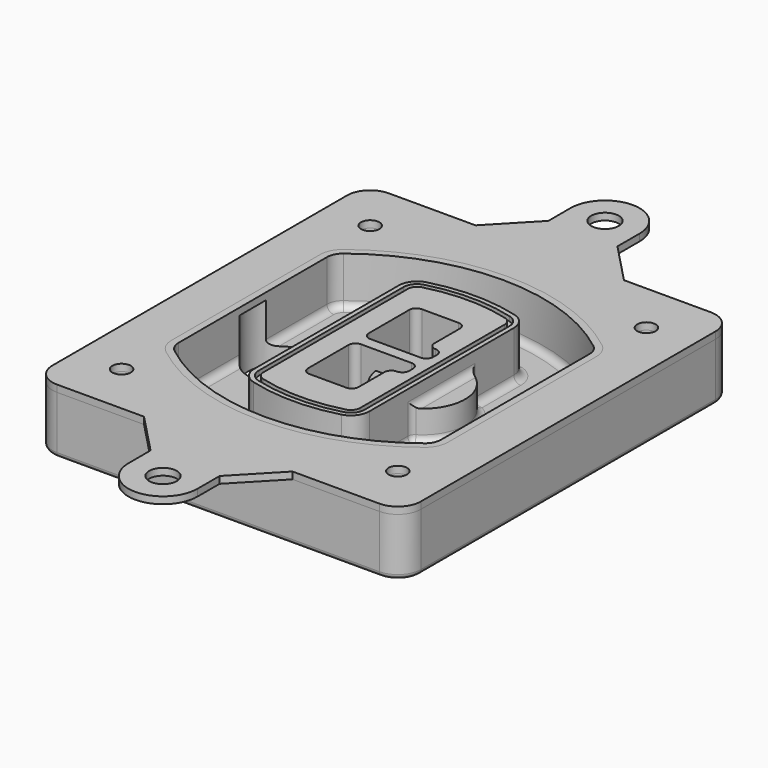
from build123d import *

# Parameters (mm, degrees)
F0_R      = 4
F1_DEPTH  = 25
F2_DEPTH  = 3
F3_DEPTH  = 18
F5_DEPTH  = 21
F6_DEPTH  = 2
F8_DEPTH  = 20
F9_DEPTH  = 16
F10_DEPTH = 25
F7_R      = 6
F7_R_2    = 4
F11_DEPTH = 6
F13_DEPTH = 9
F14_R     = 3
F15_R     = 2
F16_R     = 6
F16_R_2   = 4
F17_DEPTH = 3


with BuildPart() as f1:
    # F0 (on Top) → F1 (new body)
    with BuildSketch(Plane.XY):
        with BuildLine():
            ThreePointArc((-80, -80), (-77.0710678119, -87.0710678119), (-70, -90))
            Line((-70, -90), (70, -90))
            ThreePointArc((70, -90), (77.0710678119, -87.0710678119), (80, -80))
            Line((80, -80), (80, 80))
            ThreePointArc((80, 80), (77.0710678119, 87.0710678119), (70, 90))
            Line((70, 90), (-70, 90))
            ThreePointArc((-70, 90), (-77.0710678119, 87.0710678119), (-80, 80))
            Line((-80, 80), (-80, -80))
        make_face()
        with Locations((-60, -67.5)):
            Circle(F0_R, mode=Mode.SUBTRACT)
        with Locations((60, -67.5)):
            Circle(F0_R, mode=Mode.SUBTRACT)
        with Locations((-60, 67.5)):
            Circle(F0_R, mode=Mode.SUBTRACT)
        with BuildLine():
            ThreePointArc((-64, 40.2934422872), (-62.5820384798, 46.4328484224), (-58.6153846154, 51.3286200352))
            ThreePointArc((-58.6153846154, 51.3286200352), (0, 71.5), (58.6153846154, 51.3286200352))
            ThreePointArc((58.6153846154, 51.3286200352), (62.5820384798, 46.4328484224), (64, 40.2934422872))
            Line((64, 40.2934422872), (64, -40.2934422872))
            ThreePointArc((64, -40.2934422872), (62.5820384798, -46.4328484224), (58.6153846154, -51.3286200352))
            ThreePointArc((58.6153846154, -51.3286200352), (0, -71.5), (-58.6153846154, -51.3286200352))
            ThreePointArc((-58.6153846154, -51.3286200352), (-62.5820384798, -46.4328484224), (-64, -40.2934422872))
            Line((-64, -40.2934422872), (-64, 40.2934422872))
        make_face(mode=Mode.SUBTRACT)
        with Locations((60, 67.5)):
            Circle(F0_R, mode=Mode.SUBTRACT)
        with BuildLine():
            ThreePointArc((58.6153846154, 51.3286200352), (0, 71.5), (-58.6153846154, 51.3286200352))
            ThreePointArc((-58.6153846154, 51.3286200352), (-62.5820384798, 46.4328484224), (-64, 40.2934422872))
            Line((-64, 40.2934422872), (-64, -40.2934422872))
            ThreePointArc((-64, -40.2934422872), (-62.5820384798, -46.4328484224), (-58.6153846154, -51.3286200352))
            ThreePointArc((-58.6153846154, -51.3286200352), (0, -71.5), (58.6153846154, -51.3286200352))
            ThreePointArc((58.6153846154, -51.3286200352), (62.5820384798, -46.4328484224), (64, -40.2934422872))
            Line((64, -40.2934422872), (64, 40.2934422872))
            ThreePointArc((64, 40.2934422872), (62.5820384798, 46.4328484224), (58.6153846154, 51.3286200352))
        make_face()
        with BuildLine():
            Line((-60, -40.2934422872), (-60, 40.2934422872))
            ThreePointArc((-60, 40.2934422872), (-58.9871703427, 44.6787323838), (-56.1538461538, 48.1757121072))
            ThreePointArc((-56.1538461538, 48.1757121072), (0, 67.5), (56.1538461538, 48.1757121072))
            ThreePointArc((56.1538461538, 48.1757121072), (58.9871703427, 44.6787323838), (60, 40.2934422872))
            Line((60, 40.2934422872), (60, -40.2934422872))
            ThreePointArc((60, -40.2934422872), (58.9871703427, -44.6787323838), (56.1538461538, -48.1757121072))
            ThreePointArc((56.1538461538, -48.1757121072), (0, -67.5), (-56.1538461538, -48.1757121072))
            ThreePointArc((-56.1538461538, -48.1757121072), (-58.9871703427, -44.6787323838), (-60, -40.2934422872))
        make_face(mode=Mode.SUBTRACT)
        with BuildLine():
            ThreePointArc((-56.1538461538, 48.1757121072), (-58.9871703427, 44.6787323838), (-60, 40.2934422872))
            Line((-60, 40.2934422872), (-60, -40.2934422872))
            ThreePointArc((-60, -40.2934422872), (-58.9871703427, -44.6787323838), (-56.1538461538, -48.1757121072))
            ThreePointArc((-56.1538461538, -48.1757121072), (0, -67.5), (56.1538461538, -48.1757121072))
            ThreePointArc((56.1538461538, -48.1757121072), (58.9871703427, -44.6787323838), (60, -40.2934422872))
            Line((60, -40.2934422872), (60, 40.2934422872))
            ThreePointArc((60, 40.2934422872), (58.9871703427, 44.6787323838), (56.1538461538, 48.1757121072))
            ThreePointArc((56.1538461538, 48.1757121072), (0, 67.5), (-56.1538461538, 48.1757121072))
        make_face()
        with BuildLine():
            ThreePointArc((54.3076923077, 45.8110311612), (56.2910192399, 43.3631453548), (57, 40.2934422872))
            Line((57, 40.2934422872), (57, -40.2934422872))
            ThreePointArc((57, -40.2934422872), (56.2910192399, -43.3631453548), (54.3076923077, -45.8110311612))
            ThreePointArc((54.3076923077, -45.8110311612), (0, -64.5), (-54.3076923077, -45.8110311612))
            ThreePointArc((-54.3076923077, -45.8110311612), (-56.2910192399, -43.3631453548), (-57, -40.2934422872))
            Line((-57, -40.2934422872), (-57, 40.2934422872))
            ThreePointArc((-57, 40.2934422872), (-56.2910192399, 43.3631453548), (-54.3076923077, 45.8110311612))
            ThreePointArc((-54.3076923077, 45.8110311612), (0, 64.5), (54.3076923077, 45.8110311612))
        make_face(mode=Mode.SUBTRACT)
        with BuildLine():
            Line((57, -40.2934422872), (57, 40.2934422872))
            ThreePointArc((57, 40.2934422872), (56.2910192399, 43.3631453548), (54.3076923077, 45.8110311612))
            ThreePointArc((54.3076923077, 45.8110311612), (0, 64.5), (-54.3076923077, 45.8110311612))
            ThreePointArc((-54.3076923077, 45.8110311612), (-56.2910192399, 43.3631453548), (-57, 40.2934422872))
            Line((-57, 40.2934422872), (-57, -40.2934422872))
            ThreePointArc((-57, -40.2934422872), (-56.2910192399, -43.3631453548), (-54.3076923077, -45.8110311612))
            ThreePointArc((-54.3076923077, -45.8110311612), (0, -64.5), (54.3076923077, -45.8110311612))
            ThreePointArc((54.3076923077, -45.8110311612), (56.2910192399, -43.3631453548), (57, -40.2934422872))
        make_face()
    extrude(amount=-F1_DEPTH)

    # F0 (on Top) → F2 (join)
    with BuildSketch(Plane.XY):
        with BuildLine():
            ThreePointArc((-56.1538461538, 48.1757121072), (-58.9871703427, 44.6787323838), (-60, 40.2934422872))
            Line((-60, 40.2934422872), (-60, -40.2934422872))
            ThreePointArc((-60, -40.2934422872), (-58.9871703427, -44.6787323838), (-56.1538461538, -48.1757121072))
            ThreePointArc((-56.1538461538, -48.1757121072), (0, -67.5), (56.1538461538, -48.1757121072))
            ThreePointArc((56.1538461538, -48.1757121072), (58.9871703427, -44.6787323838), (60, -40.2934422872))
            Line((60, -40.2934422872), (60, 40.2934422872))
            ThreePointArc((60, 40.2934422872), (58.9871703427, 44.6787323838), (56.1538461538, 48.1757121072))
            ThreePointArc((56.1538461538, 48.1757121072), (0, 67.5), (-56.1538461538, 48.1757121072))
        make_face()
        with BuildLine():
            ThreePointArc((54.3076923077, 45.8110311612), (56.2910192399, 43.3631453548), (57, 40.2934422872))
            Line((57, 40.2934422872), (57, -40.2934422872))
            ThreePointArc((57, -40.2934422872), (56.2910192399, -43.3631453548), (54.3076923077, -45.8110311612))
            ThreePointArc((54.3076923077, -45.8110311612), (0, -64.5), (-54.3076923077, -45.8110311612))
            ThreePointArc((-54.3076923077, -45.8110311612), (-56.2910192399, -43.3631453548), (-57, -40.2934422872))
            Line((-57, -40.2934422872), (-57, 40.2934422872))
            ThreePointArc((-57, 40.2934422872), (-56.2910192399, 43.3631453548), (-54.3076923077, 45.8110311612))
            ThreePointArc((-54.3076923077, 45.8110311612), (0, 64.5), (54.3076923077, 45.8110311612))
        make_face(mode=Mode.SUBTRACT)
    extrude(amount=F2_DEPTH)

    # F0 (on Top) → F3 (cut)
    with BuildSketch(Plane.XY):
        with BuildLine():
            Line((57, -40.2934422872), (57, 40.2934422872))
            ThreePointArc((57, 40.2934422872), (56.2910192399, 43.3631453548), (54.3076923077, 45.8110311612))
            ThreePointArc((54.3076923077, 45.8110311612), (0, 64.5), (-54.3076923077, 45.8110311612))
            ThreePointArc((-54.3076923077, 45.8110311612), (-56.2910192399, 43.3631453548), (-57, 40.2934422872))
            Line((-57, 40.2934422872), (-57, -40.2934422872))
            ThreePointArc((-57, -40.2934422872), (-56.2910192399, -43.3631453548), (-54.3076923077, -45.8110311612))
            ThreePointArc((-54.3076923077, -45.8110311612), (0, -64.5), (54.3076923077, -45.8110311612))
            ThreePointArc((54.3076923077, -45.8110311612), (56.2910192399, -43.3631453548), (57, -40.2934422872))
        make_face()
    extrude(amount=-F3_DEPTH, mode=Mode.SUBTRACT)

    # F4 (on face) → F5 (join, through all)
    with BuildSketch(Plane.XY.offset(3)):
        with BuildLine():
            ThreePointArc((-25, -39.2465276821), (-23.3511545998, -44.1109737193), (-19.0842911877, -46.9702398883))
            ThreePointArc((-19.0842911877, -46.9702398883), (0, -49.5), (19.0842911877, -46.9702398883))
            ThreePointArc((19.0842911877, -46.9702398883), (23.3511545998, -44.1109737193), (25, -39.2465276821))
            Line((25, -39.2465276821), (25, 39.2465276821))
            ThreePointArc((25, 39.2465276821), (23.3511545998, 44.1109737193), (19.0842911877, 46.9702398883))
            ThreePointArc((19.0842911877, 46.9702398883), (0, 49.5), (-19.0842911877, 46.9702398883))
            ThreePointArc((-19.0842911877, 46.9702398883), (-23.3511545998, 44.1109737193), (-25, 39.2465276821))
            Line((-25, 39.2465276821), (-25, -39.2465276821))
        make_face()
        with BuildLine():
            ThreePointArc((18.5632183908, 45.0393118368), (21.7633659499, 42.89486221), (23, 39.2465276821))
            Line((23, 39.2465276821), (23, -39.2465276821))
            ThreePointArc((23, -39.2465276821), (21.7633659499, -42.89486221), (18.5632183908, -45.0393118368))
            ThreePointArc((18.5632183908, -45.0393118368), (0, -47.5), (-18.5632183908, -45.0393118368))
            ThreePointArc((-18.5632183908, -45.0393118368), (-21.7633659499, -42.89486221), (-23, -39.2465276821))
            Line((-23, -39.2465276821), (-23, 39.2465276821))
            ThreePointArc((-23, 39.2465276821), (-21.7633659499, 42.89486221), (-18.5632183908, 45.0393118368))
            ThreePointArc((-18.5632183908, 45.0393118368), (0, 47.5), (18.5632183908, 45.0393118368))
        make_face(mode=Mode.SUBTRACT)
        with BuildLine():
            Line((23, -39.2465276821), (23, 39.2465276821))
            ThreePointArc((23, 39.2465276821), (21.7633659499, 42.89486221), (18.5632183908, 45.0393118368))
            ThreePointArc((18.5632183908, 45.0393118368), (0, 47.5), (-18.5632183908, 45.0393118368))
            ThreePointArc((-18.5632183908, 45.0393118368), (-21.7633659499, 42.89486221), (-23, 39.2465276821))
            Line((-23, 39.2465276821), (-23, -39.2465276821))
            ThreePointArc((-23, -39.2465276821), (-21.7633659499, -42.89486221), (-18.5632183908, -45.0393118368))
            ThreePointArc((-18.5632183908, -45.0393118368), (0, -47.5), (18.5632183908, -45.0393118368))
            ThreePointArc((18.5632183908, -45.0393118368), (21.7633659499, -42.89486221), (23, -39.2465276821))
        make_face()
        with BuildLine():
            ThreePointArc((18.0421455939, 43.1083837852), (20.1755772999, 41.6787507007), (21, 39.2465276821))
            Line((21, 39.2465276821), (21, -39.2465276821))
            ThreePointArc((21, -39.2465276821), (20.1755772999, -41.6787507007), (18.0421455939, -43.1083837852))
            ThreePointArc((18.0421455939, -43.1083837852), (0, -45.5), (-18.0421455939, -43.1083837852))
            ThreePointArc((-18.0421455939, -43.1083837852), (-20.1755772999, -41.6787507007), (-21, -39.2465276821))
            Line((-21, -39.2465276821), (-21, 39.2465276821))
            ThreePointArc((-21, 39.2465276821), (-20.1755772999, 41.6787507007), (-18.0421455939, 43.1083837852))
            ThreePointArc((-18.0421455939, 43.1083837852), (0, 45.5), (18.0421455939, 43.1083837852))
        make_face(mode=Mode.SUBTRACT)
        with BuildLine():
            Line((21, -39.2465276821), (21, 39.2465276821))
            ThreePointArc((21, 39.2465276821), (20.1755772999, 41.6787507007), (18.0421455939, 43.1083837852))
            ThreePointArc((18.0421455939, 43.1083837852), (0, 45.5), (-18.0421455939, 43.1083837852))
            ThreePointArc((-18.0421455939, 43.1083837852), (-20.1755772999, 41.6787507007), (-21, 39.2465276821))
            Line((-21, 39.2465276821), (-21, -39.2465276821))
            ThreePointArc((-21, -39.2465276821), (-20.1755772999, -41.6787507007), (-18.0421455939, -43.1083837852))
            ThreePointArc((-18.0421455939, -43.1083837852), (0, -45.5), (18.0421455939, -43.1083837852))
            ThreePointArc((18.0421455939, -43.1083837852), (20.1755772999, -41.6787507007), (21, -39.2465276821))
        make_face()
        with BuildLine():
            Line((-8, -2.5), (14, -2.5))
            ThreePointArc((14, -2.5), (16.1213203436, -3.3786796564), (17, -5.5))
            Line((17, -5.5), (17, -7.5))
            ThreePointArc((17, -7.5), (16.1213203436, -9.6213203436), (14, -10.5))
            ThreePointArc((14, -10.5), (11.8786796564, -11.3786796564), (11, -13.5))
            Line((11, -13.5), (11, -27.5))
            ThreePointArc((11, -27.5), (10.1213203436, -29.6213203436), (8, -30.5))
            Line((8, -30.5), (-8, -30.5))
            ThreePointArc((-8, -30.5), (-10.1213203436, -29.6213203436), (-11, -27.5))
            Line((-11, -27.5), (-11, -5.5))
            ThreePointArc((-11, -5.5), (-10.1213203436, -3.3786796564), (-8, -2.5))
        make_face(mode=Mode.SUBTRACT)
        with BuildLine():
            ThreePointArc((-8, 2.5), (-10.1213203436, 3.3786796564), (-11, 5.5))
            Line((-11, 5.5), (-11, 27.5))
            ThreePointArc((-11, 27.5), (-10.1213203436, 29.6213203436), (-8, 30.5))
            Line((-8, 30.5), (8, 30.5))
            ThreePointArc((8, 30.5), (10.1213203436, 29.6213203436), (11, 27.5))
            Line((11, 27.5), (11, 13.5))
            ThreePointArc((11, 13.5), (11.8786796564, 11.3786796564), (14, 10.5))
            ThreePointArc((14, 10.5), (16.1213203436, 9.6213203436), (17, 7.5))
            Line((17, 7.5), (17, 5.5))
            ThreePointArc((17, 5.5), (16.1213203436, 3.3786796564), (14, 2.5))
            Line((14, 2.5), (-8, 2.5))
        make_face(mode=Mode.SUBTRACT)
    extrude(amount=-F5_DEPTH)

    # F4 (on face) → F6 (cut)
    with BuildSketch(Plane.XY.offset(3)):
        with BuildLine():
            Line((23, -39.2465276821), (23, 39.2465276821))
            ThreePointArc((23, 39.2465276821), (21.7633659499, 42.89486221), (18.5632183908, 45.0393118368))
            ThreePointArc((18.5632183908, 45.0393118368), (0, 47.5), (-18.5632183908, 45.0393118368))
            ThreePointArc((-18.5632183908, 45.0393118368), (-21.7633659499, 42.89486221), (-23, 39.2465276821))
            Line((-23, 39.2465276821), (-23, -39.2465276821))
            ThreePointArc((-23, -39.2465276821), (-21.7633659499, -42.89486221), (-18.5632183908, -45.0393118368))
            ThreePointArc((-18.5632183908, -45.0393118368), (0, -47.5), (18.5632183908, -45.0393118368))
            ThreePointArc((18.5632183908, -45.0393118368), (21.7633659499, -42.89486221), (23, -39.2465276821))
        make_face()
        with BuildLine():
            ThreePointArc((18.0421455939, 43.1083837852), (20.1755772999, 41.6787507007), (21, 39.2465276821))
            Line((21, 39.2465276821), (21, -39.2465276821))
            ThreePointArc((21, -39.2465276821), (20.1755772999, -41.6787507007), (18.0421455939, -43.1083837852))
            ThreePointArc((18.0421455939, -43.1083837852), (0, -45.5), (-18.0421455939, -43.1083837852))
            ThreePointArc((-18.0421455939, -43.1083837852), (-20.1755772999, -41.6787507007), (-21, -39.2465276821))
            Line((-21, -39.2465276821), (-21, 39.2465276821))
            ThreePointArc((-21, 39.2465276821), (-20.1755772999, 41.6787507007), (-18.0421455939, 43.1083837852))
            ThreePointArc((-18.0421455939, 43.1083837852), (0, 45.5), (18.0421455939, 43.1083837852))
        make_face(mode=Mode.SUBTRACT)
    extrude(amount=-F6_DEPTH, mode=Mode.SUBTRACT)

    # F7 (on face) → F8 (join)
    with BuildSketch(Plane(origin=(0, 0, -25), x_dir=(1, 0, 0), z_dir=(0, 0, -1))):
        with BuildLine():
            ThreePointArc((3.28842436, 0), (16.7567035675, 13.4682792075), (30.224982775, 0))
            Line((30.224982775, 0), (35.224982775, 0))
            ThreePointArc((35.224982775, 0), (16.7567035675, 18.4682792075), (-1.71157564, 0))
            Line((-1.71157564, 0), (3.28842436, 0))
        make_face()
        with BuildLine():
            Line((3.28842436, 0), (30.224982775, 0))
            ThreePointArc((30.224982775, 0), (16.7567035675, 13.4682792075), (3.28842436, 0))
        make_face()
        with BuildLine():
            ThreePointArc((3.28842436, 0), (16.7567035675, -13.4682792075), (30.224982775, 0))
            Line((30.224982775, 0), (3.28842436, 0))
        make_face()
        with BuildLine():
            Line((35.224982775, 0), (30.224982775, 0))
            ThreePointArc((30.224982775, 0), (16.7567035675, -13.4682792075), (3.28842436, 0))
            Line((3.28842436, 0), (-1.71157564, 0))
            ThreePointArc((-1.71157564, 0), (16.7567035675, -18.4682792075), (35.224982775, 0))
        make_face()
    extrude(amount=-F8_DEPTH)

    # F7 (on face) → F9 (cut)
    with BuildSketch(Plane(origin=(0, 0, -25), x_dir=(1, 0, 0), z_dir=(0, 0, -1))):
        with BuildLine():
            Line((3.28842436, 0), (30.224982775, 0))
            ThreePointArc((30.224982775, 0), (16.7567035675, 13.4682792075), (3.28842436, 0))
        make_face()
        with BuildLine():
            ThreePointArc((3.28842436, 0), (16.7567035675, -13.4682792075), (30.224982775, 0))
            Line((30.224982775, 0), (3.28842436, 0))
        make_face()
    extrude(amount=-F9_DEPTH, mode=Mode.SUBTRACT)

    # F7 (on face) → F10 (cut)
    with BuildSketch(Plane(origin=(0, 0, -25), x_dir=(1, 0, 0), z_dir=(0, 0, -1))):
        with BuildLine():
            Line((-59.0318229325, 0), (-32.0952645175, 0))
            ThreePointArc((-32.0952645175, 0), (-45.563543725, 13.4682792075), (-59.0318229325, 0))
        make_face()
        with BuildLine():
            ThreePointArc((-59.0318229325, 0), (-45.563543725, -13.4682792075), (-32.0952645175, 0))
            Line((-32.0952645175, 0), (-59.0318229325, 0))
        make_face()
    extrude(amount=-F10_DEPTH, mode=Mode.SUBTRACT)

    # F7 (on face) → F11 (cut)
    with BuildSketch(Plane(origin=(0, 0, -25), x_dir=(1, 0, 0), z_dir=(0, 0, -1))):
        with Locations((60, -67.5)):
            Circle(F7_R)
        with Locations((60, -67.5)):
            Circle(F7_R_2, mode=Mode.SUBTRACT)
        with Locations((-60, -67.5)):
            Circle(F7_R)
        with Locations((-60, -67.5)):
            Circle(F7_R_2, mode=Mode.SUBTRACT)
        with Locations((-60, 67.5)):
            Circle(F7_R)
        with Locations((-60, 67.5)):
            Circle(F7_R_2, mode=Mode.SUBTRACT)
        with Locations((60, 67.5)):
            Circle(F7_R)
        with Locations((60, 67.5)):
            Circle(F7_R_2, mode=Mode.SUBTRACT)
    extrude(amount=-F11_DEPTH, mode=Mode.SUBTRACT)

    # F12 (on face) → F13 (cut, through all)
    with BuildSketch(Plane(origin=(0, 0, -9), x_dir=(1, 0, 0), z_dir=(0, 0, -1))):
        with BuildLine():
            Line((11, 13.5), (11, 17.5481537753))
            ThreePointArc((11, 17.5481537753), (2.5696536419, 11.8239143813), (-1.5415842455, 2.5))
            Line((-1.5415842455, 2.5), (3.5224848595, 2.5))
            ThreePointArc((3.5224848595, 2.5), (6.1857188154, 8.3455872281), (11.2536447004, 12.2927168648))
            ThreePointArc((11.2536447004, 12.2927168648), (11.0640958889, 12.8831798879), (11, 13.5))
        make_face()
        with BuildLine():
            ThreePointArc((11.2536447004, -12.2927168648), (6.1857188154, -8.3455872281), (3.5224848595, -2.5))
            Line((3.5224848595, -2.5), (-1.5415842455, -2.5))
            ThreePointArc((-1.5415842455, -2.5), (2.5696536419, -11.8239143813), (11, -17.5481537753))
            Line((11, -17.5481537753), (11, -13.5))
            ThreePointArc((11, -13.5), (11.0640958889, -12.8831798879), (11.2536447004, -12.2927168648))
        make_face()
        with BuildLine():
            ThreePointArc((11.2536447004, 12.2927168648), (6.1857188154, 8.3455872281), (3.5224848595, 2.5))
            Line((3.5224848595, 2.5), (14, 2.5))
            ThreePointArc((14, 2.5), (16.1213203436, 3.3786796564), (17, 5.5))
            Line((17, 5.5), (17, 7.5))
            ThreePointArc((17, 7.5), (16.1213203436, 9.6213203436), (14, 10.5))
            ThreePointArc((14, 10.5), (12.3601599782, 10.9878446101), (11.2536447004, 12.2927168648))
        make_face()
        with BuildLine():
            Line((14, -2.5), (3.5224848595, -2.5))
            ThreePointArc((3.5224848595, -2.5), (6.1857188154, -8.3455872281), (11.2536447004, -12.2927168648))
            ThreePointArc((11.2536447004, -12.2927168648), (12.3601599782, -10.9878446101), (14, -10.5))
            ThreePointArc((14, -10.5), (16.1213203436, -9.6213203436), (17, -7.5))
            Line((17, -7.5), (17, -5.5))
            ThreePointArc((17, -5.5), (16.1213203436, -3.3786796564), (14, -2.5))
        make_face()
    extrude(amount=F13_DEPTH, mode=Mode.SUBTRACT)

    # F14
    f14_edges = [f1.edges().sort_by_distance(p)[0] for p in [
        (-57, -23.703476, -18),
        (-57, 23.703476, -18),
        (25, 0, -5),
        (25, 16.526506, -11.5),
        (25, -16.526506, -11.5),
        (25, -27.886517, -18),
        (35.224983, 0, -18),
    ]]
    fillet(f14_edges, radius=F14_R)

    # F15
    f15_edges = [f1.edges().sort_by_distance(p)[0] for p in [
        (0, -90, -25),
    ]]
    fillet(f15_edges, radius=F15_R)


with BuildPart() as f17:
    # F16 (on face) → F17 (new body, through all)
    with BuildSketch(Plane.XY):
        with BuildLine():
            Line((-32.2395451367, -90), (-15, -108))
            Line((-15, -108), (-15, -120))
            ThreePointArc((-15, -120), (0, -135), (15, -120))
            Line((15, -120), (15, -108))
            Line((15, -108), (32.2395451367, -90))
            Line((32.2395451367, -90), (-32.2395451367, -90))
        make_face()
        with Locations((0, -120)):
            Circle(F16_R, mode=Mode.SUBTRACT)
        with BuildLine():
            Line((32.2395451367, 90), (-32.2395451367, 90))
            Line((-32.2395451367, 90), (-33, 90))
            Line((-33, 90), (-70, 90))
            ThreePointArc((-70, 90), (-77.0710678119, 87.0710678119), (-80, 80))
            Line((-80, 80), (-80, -80))
            ThreePointArc((-80, -80), (-77.0710678119, -87.0710678119), (-70, -90))
            Line((-70, -90), (-33, -90))
            Line((-33, -90), (-32.2395451367, -90))
            Line((-32.2395451367, -90), (32.2395451367, -90))
            Line((32.2395451367, -90), (33, -90))
            Line((33, -90), (70, -90))
            ThreePointArc((70, -90), (77.0710678119, -87.0710678119), (80, -80))
            Line((80, -80), (80, 80))
            ThreePointArc((80, 80), (77.0710678119, 87.0710678119), (70, 90))
            Line((70, 90), (33, 90))
            Line((33, 90), (32.2395451367, 90))
        make_face()
        with Locations((-60, -67.5)):
            Circle(F16_R_2, mode=Mode.SUBTRACT)
        with Locations((60, -67.5)):
            Circle(F16_R_2, mode=Mode.SUBTRACT)
        with Locations((-60, 67.5)):
            Circle(F16_R_2, mode=Mode.SUBTRACT)
        with BuildLine():
            ThreePointArc((-60, 40.2934422872), (-58.9871703427, 44.6787323838), (-56.1538461538, 48.1757121072))
            ThreePointArc((-56.1538461538, 48.1757121072), (0, 67.5), (56.1538461538, 48.1757121072))
            ThreePointArc((56.1538461538, 48.1757121072), (58.9871703427, 44.6787323838), (60, 40.2934422872))
            Line((60, 40.2934422872), (60, -40.2934422872))
            ThreePointArc((60, -40.2934422872), (58.9871703427, -44.6787323838), (56.1538461538, -48.1757121072))
            ThreePointArc((56.1538461538, -48.1757121072), (0, -67.5), (-56.1538461538, -48.1757121072))
            ThreePointArc((-56.1538461538, -48.1757121072), (-58.9871703427, -44.6787323838), (-60, -40.2934422872))
            Line((-60, -40.2934422872), (-60, 40.2934422872))
        make_face(mode=Mode.SUBTRACT)
        with Locations((60, 67.5)):
            Circle(F16_R_2, mode=Mode.SUBTRACT)
        with BuildLine():
            Line((-15, 108), (-32.2395451367, 90))
            Line((-32.2395451367, 90), (32.2395451367, 90))
            Line((32.2395451367, 90), (15, 108))
            Line((15, 108), (15, 120))
            ThreePointArc((15, 120), (0, 135), (-15, 120))
            Line((-15, 120), (-15, 108))
        make_face()
        with Locations((0, 120)):
            Circle(F16_R, mode=Mode.SUBTRACT)
    extrude(amount=F17_DEPTH)


solid = Compound([f1.part, f17.part])
